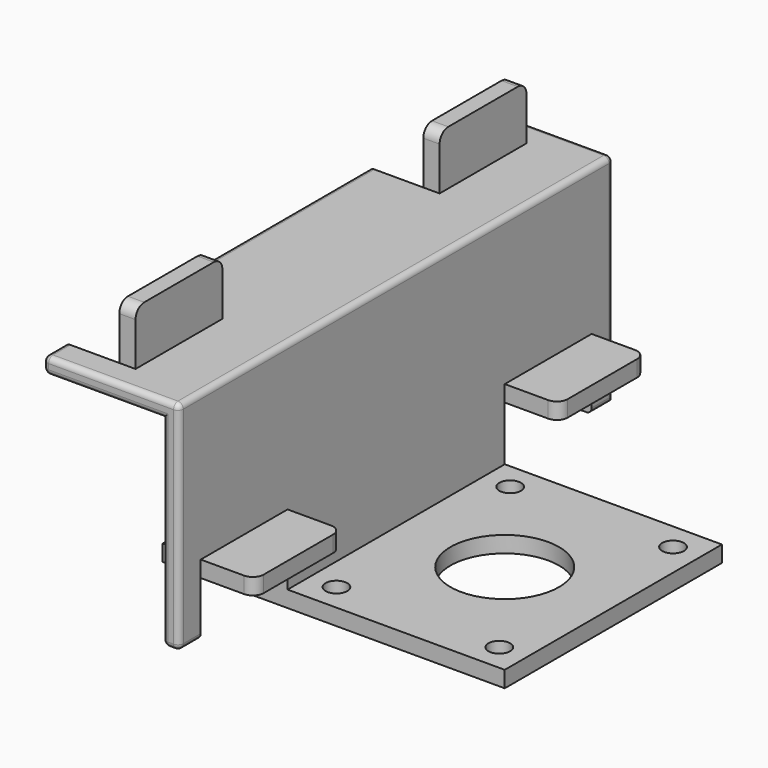
from build123d import *

# Parameters (mm, degrees)
F1_DEPTH      = 50
F2_W          = 20
F2_H          = 10
F3_DEPTH      = 3
F2_H_2        = 3
F4_DEPTH      = 10
F5_W          = 10
F5_H          = 20
F6_DEPTH      = 3
F5_W_2        = 3
F7_DEPTH      = 10
F8_R          = 2
F9_R          = 1
F10_R         = 1
F11_R         = 1
F12_T1_DEPTH  = 98
F12_S5_W      = 1
F12_S5_H      = 1
F12_T6_DEPTH  = 1
F12_S11_W     = 1
F12_S11_H     = 1
F12_T12_DEPTH = 1
F13_W         = 50
F13_H         = 3
F14_DEPTH     = 23
F15_W         = 50
F15_H         = 3
F16_DEPTH     = 40
F17_R         = 2
F17_R_2       = 10
F18_DEPTH     = 25


# Not quite as in the source:
# - a fillet or chamfer that OpenCascade refuses, or shapes differently, is made with other operations: its cross-section is extruded or revolved along the edge and cut away or added


with BuildPart() as f1:
    # F0 (on Front) → F1 (new body, symmetric)
    with BuildSketch(Plane.XZ):
        Polygon((-3, 0), (0, 0), (0, 40), (-25, 40), (-25, 37), (-3, 37), align=None)
    extrude(amount=F1_DEPTH, both=True)

    # F2 (on face) → F3 (cut, through all)
    with BuildSketch(Plane.YZ):
        with Locations((-35, 5)):
            Rectangle(F2_W, F2_H)
        with Locations((35, 5)):
            Rectangle(F2_W, F2_H)
    extrude(amount=-F3_DEPTH, mode=Mode.SUBTRACT)

    # F2 (on face) → F4 (join)
    with BuildSketch(Plane.YZ):
        with Locations((-35, 11.5)):
            Rectangle(F2_W, F2_H_2)
        with Locations((35, 11.5)):
            Rectangle(F2_W, F2_H_2)
    extrude(amount=F4_DEPTH)

    # F5 (on face) → F6 (cut, through all)
    with BuildSketch(Plane.XY.offset(40)):
        with Locations((-20, 35)):
            Rectangle(F5_W, F5_H)
        with Locations((-20, -35)):
            Rectangle(F5_W, F5_H)
    extrude(amount=-F6_DEPTH, mode=Mode.SUBTRACT)

    # F5 (on face) → F7 (join)
    with BuildSketch(Plane.XY.offset(40)):
        with Locations((-13.5, 35)):
            Rectangle(F5_W_2, F5_H)
        with Locations((-13.5, -35)):
            Rectangle(F5_W_2, F5_H)
    extrude(amount=F7_DEPTH)

    # F8
    f8_edges = [f1.edges().sort_by_distance(p)[0] for p in [
        (-13.5, 25, 50),
        (-13.5, 45, 50),
        (-13.5, -25, 50),
        (-13.5, -45, 50),
        (10, -45, 11.5),
        (10, -25, 11.5),
        (10, 25, 11.5),
        (10, 45, 11.5),
    ]]
    fillet(f8_edges, radius=F8_R)

    # F9
    f9_edges = [f1.edges().sort_by_distance(p)[0] for p in [
        (-12.5, -50, 40),
        (0, -50, 20),
        (-3, -50, 18.5),
        (-14, -50, 37),
    ]]
    fillet(f9_edges, radius=F9_R)

    # F10
    f10_edges = [f1.edges().sort_by_distance(p)[0] for p in [
        (-25, -47, 37),
        (-25, -47, 40),
    ]]
    fillet(f10_edges, radius=F10_R)

    # F11
    f11_edges = [f1.edges().sort_by_distance(p)[0] for p in [
        (-25, 0, 40),
        (-25, 0, 37),
        (-25, 47.5, 40),
        (-25, 47.5, 37),
        (-14, 50, 37),
        (-12.5, 50, 40),
        (-3, 50, 18.5),
        (0, 50, 20),
        (-3, 47.5, 0),
        (0, 47.5, 0),
        (-3, -47, 0),
        (0, -47, 0),
    ]]
    fillet(f11_edges, radius=F11_R)

    # F12: fillet of radius 1 on 1 edges, made by hand

    # F12_s2 → F12_t1 (cut)
    with BuildSketch(Plane.XZ.offset(-49)):
        with BuildLine():
            ThreePointArc((-1, 40), (-0.2928932188, 39.7071067812), (0, 39))
            Line((0, 39), (0, 40))
            Line((0, 40), (-1, 40))
        make_face()
    extrude(amount=F12_T1_DEPTH, mode=Mode.SUBTRACT)


with BuildPart() as f12_tool4:
    # F12_s5 → F12_t6 (new body)
    with BuildSketch(Plane.XY.offset(39)):
        with Locations((-0.5, 49.5)):
            Rectangle(F12_S5_W, F12_S5_H)
    extrude(amount=F12_T6_DEPTH)

    # F12_s7 → F12_t8 (revolve, cut)
    with BuildSketch(Plane(origin=(-1, 49, 39), x_dir=(-0.7071067812, -0.7071067812, 0), z_dir=(-0.7071067812, 0.7071067812, 0))):
        with BuildLine():
            ThreePointArc((0, -1), (1, 0), (0, 1))
            Line((0, 1), (0, -1))
        make_face()
    revolve(axis=Axis((-1, 49, 39), (0, 0, 1)), mode=Mode.SUBTRACT)


with BuildPart() as f1_1:
    add(f1.part)

    # F12_t3: cut F12_tool4
    add(f12_tool4.part, mode=Mode.SUBTRACT)


with BuildPart() as f12_tool10:
    # F12_s11 → F12_t12 (new body)
    with BuildSketch(Plane.XY.offset(39)):
        with Locations((-0.5, -49.5)):
            Rectangle(F12_S11_W, F12_S11_H)
    extrude(amount=F12_T12_DEPTH)

    # F12_s13 → F12_t14 (revolve, cut)
    with BuildSketch(Plane(origin=(-1, -49, 39), x_dir=(-0.7071067812, 0.7071067812, 0), z_dir=(0.7071067812, 0.7071067812, 0))):
        with BuildLine():
            ThreePointArc((0, -1), (1, 0), (0, 1))
            Line((0, 1), (0, -1))
        make_face()
    revolve(axis=Axis((-1, -49, 39), (0, 0, 1)), mode=Mode.SUBTRACT)


with BuildPart() as f1_2:
    add(f1_1.part)

    # F12_t9: cut F12_tool10
    add(f12_tool10.part, mode=Mode.SUBTRACT)

    # F13 (on Right) → F14 (join)
    with BuildSketch(Plane.YZ):
        with Locations((0, -1.5)):
            Rectangle(F13_W, F13_H)
    extrude(amount=-F14_DEPTH)

    # F15 (on face) → F16 (join)
    with BuildSketch(Plane.YZ):
        with Locations((0, -1.5)):
            Rectangle(F15_W, F15_H)
    extrude(amount=F16_DEPTH)

    # F17 (on face) → F18 (cut)
    with BuildSketch(Plane(origin=(0, 0, -3), x_dir=(1, 0, 0), z_dir=(0, 0, -1))):
        with Locations((35, 20)):
            Circle(F17_R)
        with Locations((5, 20)):
            Circle(F17_R)
        with Locations((20, 0)):
            Circle(F17_R_2)
        with Locations((35, -20)):
            Circle(F17_R)
        with Locations((5, -20)):
            Circle(F17_R)
    extrude(amount=-F18_DEPTH, mode=Mode.SUBTRACT)


solid = f1_2.part
